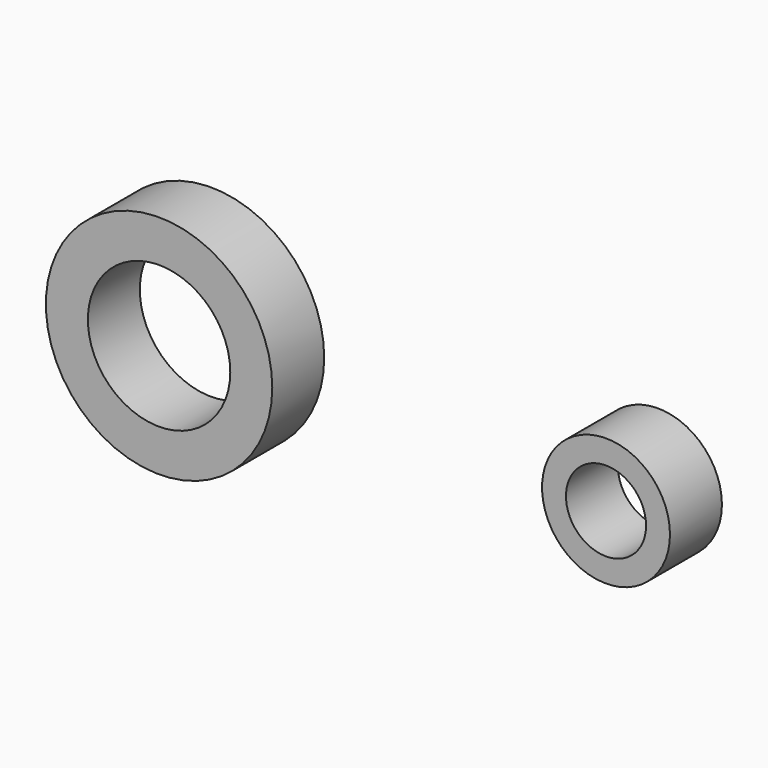
from build123d import *

# Parameters (mm, degrees)
F0_R     = 44.2728282083
F0_R_2   = 27.8473949091
F1_DEPTH = 25.4
F2_R     = 25.0148515276
F2_R_2   = 15.6616777409
F3_DEPTH = 25.4


# Not quite as in the source:
# - the program builds the solid bodies; features that only make, move or delete a surface that nothing else refers to are left out


with BuildPart() as f1:
    # F0 (on Front) → F1 (new body)
    with BuildSketch(Plane.XZ):
        with Locations((-57.833313942, 0)):
            Circle(F0_R)
        with Locations((-57.833313942, 0)):
            Circle(F0_R_2, mode=Mode.SUBTRACT)
    extrude(amount=F1_DEPTH)


with BuildPart() as f3:
    # F2 (on Front) → F3 (new body)
    with BuildSketch(Plane.XZ):
        with Locations((116.9711351395, 0)):
            Circle(F2_R)
        with Locations((116.9711351395, 0)):
            Circle(F2_R_2, mode=Mode.SUBTRACT)
    extrude(amount=F3_DEPTH)


solid = Compound([f1.part, f3.part])
